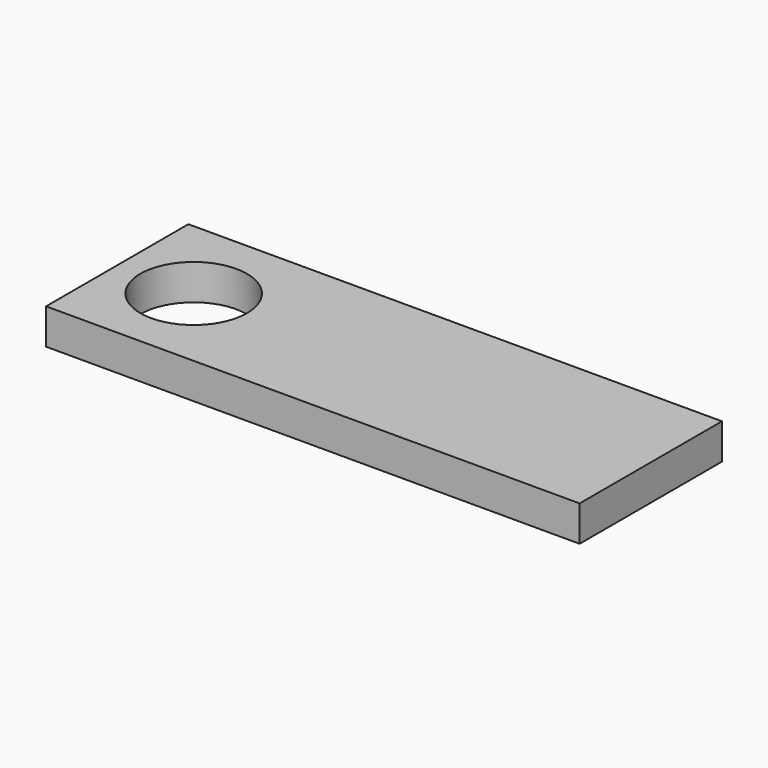
from build123d import *

# Parameters (mm, degrees)
F0_W         = 38.1
F0_H         = 12.7
F1_DEPTH     = 2.54
F2_R         = 3.81
F3_DEPTH     = 25.4
F4_TEXT_SIZE = 8.3943337409
F5_DEPTH     = 1.27


# Not quite as in the source:
# - Text() gives the source's letters only with a copy of the font that has no kerning and outlines rounded to 1/6400 em; it was checked with that copy


with BuildPart() as f1:
    # F0 (on Top) → F1 (new body)
    with BuildSketch(Plane.XY):
        with Locations((-116.8061761022, 22.2866734654)):
            Rectangle(F0_W, F0_H)
    extrude(amount=F1_DEPTH)

    # F2 (on face) → F3 (cut)
    with BuildSketch(Plane.XY.offset(2.54)):
        with Locations((-130.3978722215, 22.2866734654)):
            Circle(F2_R)
    extrude(amount=-F3_DEPTH, mode=Mode.SUBTRACT)

    # F4 (on face) → F5 (join)
    with BuildSketch(Plane.XY.offset(2.54)):
        with Locations((-123.4074383974, 19.1390831023)):
            Text('Josh', F4_TEXT_SIZE, font='Open Sans', text_align=(TextAlign.LEFT, TextAlign.BOTTOM))
    extrude(amount=-F5_DEPTH)


solid = f1.part
